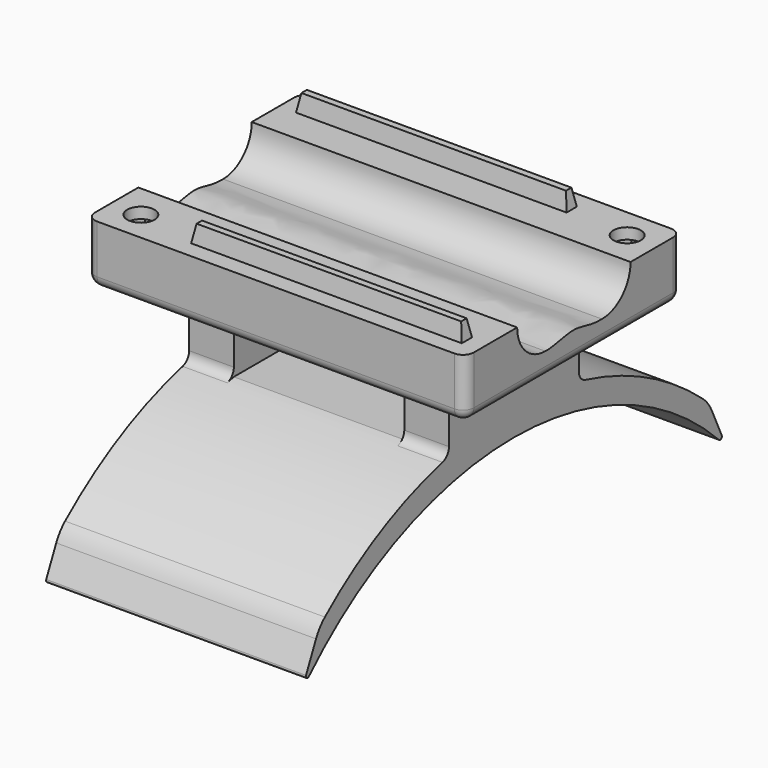
from build123d import *

# Parameters (mm, degrees)
F1_W          = 44.45
F1_H          = 31.75
F2_DEPTH      = 6.985
F4_DEPTH      = 44.45
F6_DEPTH      = 15.24
F6_DEPTH_BACK = 15.24
F7_W          = 20
F7_H          = 8.0811108913
F8_DEPTH      = 25.4
F9_R          = 1.6
F10_DEPTH     = 25.4
F11_R         = 1.6
F12_DEPTH     = 5.7
F13_W         = 31.75
F13_H         = 1.5
F14_DEPTH     = 2
F14_TAPER     = 10
F15_F1_R      = 0.254
F15_F2_R      = 0.254
F16_R         = 5.08
F18_R         = 1.27
F19_T1_DEPTH  = 5.24
F19_T3_DEPTH  = 5.24
F19_T5_DEPTH  = 8.89
F19_T7_DEPTH  = 29.21
F19_T9_DEPTH  = 41.91
F19_S13_W     = 1.2954
F19_S13_H     = 1.2954
F19_T14_DEPTH = 1.2954
F19_S19_W     = 1.2954
F19_S19_H     = 1.2954
F19_T20_DEPTH = 1.2954
F19_S25_W     = 1.2954
F19_S25_H     = 1.2954
F19_T26_DEPTH = 1.2954
F19_S31_W     = 1.2954
F19_S31_H     = 1.2954
F19_T32_DEPTH = 1.2954


# Not quite as in the source:
# - a fillet or chamfer that OpenCascade refuses, or shapes differently, is made with other operations: its cross-section is extruded or revolved along the edge and cut away or added
# - a feature of the source that left no trace in its solid (it failed there, or was rolled back) is left out


with BuildPart() as f2:
    # F1 (on Top) → F2 (new body)
    with BuildSketch(Plane.XY):
        Rectangle(F1_W, F1_H)
    extrude(amount=-F2_DEPTH)

    # F3 (on face) → F4 (cut, through all)
    with BuildSketch(Plane.YZ.offset(22.225)):
        with BuildLine():
            add(Edge.make_bspline(
                [(-4.125, 4.125), (-2.4255892558, 4.1137489608), (-0.0276085061, 2.971292738), (2.5249406681, 4.1137612248), (4.191, 4.191)],
                knots=[0, 0, 0, 0, 0.4977710734, 1, 1, 1, 1], degree=3))
            ThreePointArc((-4.125, 4.125), (-7.0418154724, 2.9168154724), (-8.25, 0))
            ThreePointArc((-8.25, 0), (-7.0418154724, -2.9168154724), (-4.125, -4.125))
            add(Edge.make_bspline(
                [(-4.125, -4.125), (-2.9335741419, -4.2006121948), (0.4172014685, -3.0581585459), (2.1438994445, -4.2006121948), (4.191, -4.191)],
                knots=[0, 0, 0, 0, 0.497799261, 1, 1, 1, 1], degree=3))
            ThreePointArc((4.191, -4.191), (7.15448452, -2.96348452), (8.382, 0))
            ThreePointArc((8.382, 0), (7.15448452, 2.96348452), (4.191, 4.191))
        make_face()
    extrude(amount=-F4_DEPTH, mode=Mode.SUBTRACT)

    # F5 (on Right) → F6 (join, two sides)
    with BuildSketch(Plane.YZ) as f6_sk:
        with BuildLine():
            ThreePointArc((-31.115, -30.5349261659), (0, -16.985), (31.115, -30.5349261659))
            Line((31.115, -30.5349261659), (28.575, -25.0251942949))
            ThreePointArc((28.575, -25.0251942949), (19.6900567688, -18.8213349574), (9.525, -15.0661108913))
            ThreePointArc((9.525, -15.0661108913), (0, -13.985), (-9.525, -15.0661108913))
            ThreePointArc((-9.525, -15.0661108913), (-19.6900567688, -18.8213349574), (-28.575, -25.0251942949))
            Line((-28.575, -25.0251942949), (-31.115, -30.5349261659))
        make_face()
        with BuildLine():
            ThreePointArc((-9.525, -15.0661108913), (0, -13.985), (9.525, -15.0661108913))
            Line((9.525, -15.0661108913), (9.525, -6.985))
            Line((9.525, -6.985), (-9.525, -6.985))
            Line((-9.525, -6.985), (-9.525, -15.0661108913))
        make_face()
    extrude(amount=F6_DEPTH)
    extrude(f6_sk.sketch, amount=-F6_DEPTH_BACK)

    # F7 (on face) → F8 (cut)
    with BuildSketch(Plane.XZ.offset(9.525)):
        with Locations((0, -11.0255554456)):
            Rectangle(F7_W, F7_H)
    extrude(amount=-F8_DEPTH, mode=Mode.SUBTRACT)

    # F9 (on face) → F10 (cut)
    with BuildSketch(Plane(origin=(0, 0, -6.985), x_dir=(1, 0, 0), z_dir=(0, 0, -1))):
        with Locations((-18.669, 12.319)):
            Circle(F9_R)
        with Locations((18.669, -12.319)):
            Circle(F9_R)
    extrude(amount=-F10_DEPTH, mode=Mode.SUBTRACT)

    # F11 (on face) → F12 (cut)
    with BuildSketch(Plane(origin=(0, 0, -6.985), x_dir=(1, 0, 0), z_dir=(0, 0, -1))):
        Polygon((-17.344, 10.02403268), (-16.019, 12.319), (-17.344, 14.61396732), (-19.994, 14.61396732), (-21.319, 12.319), (-19.994, 10.02403268), align=None)
        with Locations((-18.669, 12.319)):
            Circle(F11_R, mode=Mode.SUBTRACT)
        Polygon((19.994, -14.61396732), (21.319, -12.319), (19.994, -10.02403268), (17.344, -10.02403268), (16.019, -12.319), (17.344, -14.61396732), align=None)
        with Locations((18.669, -12.319)):
            Circle(F11_R, mode=Mode.SUBTRACT)
    extrude(amount=-F12_DEPTH, mode=Mode.SUBTRACT)

    # F13 (on face) → F14 (join)
    with BuildSketch(Plane.XY):
        with Locations((-4.35, 13.125)):
            Rectangle(F13_W, F13_H)
        with Locations((4.35, -13.125)):
            Rectangle(F13_W, F13_H)
    extrude(amount=F14_DEPTH, taper=F14_TAPER)

    # F15: fillet of radius 0.254 on 2 edges, made by hand

    # F15_f1
    f15_f1_edges = [f2.edges().sort_by_distance(p)[0] for p in [
        (0, -31.115, -30.5349261659),
    ]]
    fillet(f15_f1_edges, radius=F15_F1_R)

    # F15_f2
    f15_f2_edges = [f2.edges().sort_by_distance(p)[0] for p in [
        (0, 31.115, -30.5349261659),
    ]]
    fillet(f15_f2_edges, radius=F15_F2_R)

    # F16
    f16_edges = [f2.edges().sort_by_distance(p)[0] for p in [
        (0, 28.575, -25.025194),
        (0, -28.575, -25.025194),
    ]]
    fillet(f16_edges, radius=F16_R)

    # F18
    f18_edges = [f2.edges().sort_by_distance(p)[0] for p in [
        (12.62, 9.525, -6.985),
        (15.24, 0, -6.985),
        (12.62, -9.525, -6.985),
        (10, 0, -6.985),
        (-12.62, -9.525, -6.985),
        (-15.24, 0, -6.985),
        (-10, 0, -6.985),
        (-12.62, 9.525, -6.985),
    ]]
    fillet(f18_edges, radius=F18_R)

    # F19: fillet of radius 1.27 on 12 edges, made by hand

    # F19_s2 → F19_t1 (join)
    with BuildSketch(Plane.YZ.offset(-15.24)):
        with BuildLine():
            ThreePointArc((9.525, -14.0670689448), (9.7923311345, -14.8465271838), (10.4817797578, -15.2978382489))
            ThreePointArc((10.4817797578, -15.2978382489), (10.0040608486, -15.1792042016), (9.525, -15.0661108913))
            Line((9.525, -15.0661108913), (9.525, -14.0670689448))
        make_face()
        with BuildLine():
            ThreePointArc((-9.525, -14.0670689448), (-9.7923311345, -14.8465271838), (-10.4817797578, -15.2978382489))
            ThreePointArc((-10.4817797578, -15.2978382489), (-10.0040608486, -15.1792042016), (-9.525, -15.0661108913))
            Line((-9.525, -15.0661108913), (-9.525, -14.0670689448))
        make_face()
    extrude(amount=F19_T1_DEPTH)

    # F19_s4 → F19_t3 (join)
    with BuildSketch(Plane.YZ.offset(10)):
        with BuildLine():
            ThreePointArc((10.4817797578, -15.2978382489), (9.7923311345, -14.8465271838), (9.525, -14.0670689448))
            Line((9.525, -14.0670689448), (9.525, -15.0661108913))
            ThreePointArc((9.525, -15.0661108913), (10.0040608486, -15.1792042016), (10.4817797578, -15.2978382489))
        make_face()
        with BuildLine():
            ThreePointArc((-10.4817797578, -15.2978382489), (-9.7923311345, -14.8465271838), (-9.525, -14.0670689448))
            Line((-9.525, -14.0670689448), (-9.525, -15.0661108913))
            ThreePointArc((-9.525, -15.0661108913), (-10.0040608486, -15.1792042016), (-10.4817797578, -15.2978382489))
        make_face()
    extrude(amount=F19_T3_DEPTH)

    # F19_s6 → F19_t5 (cut)
    with BuildSketch(Plane.XY.offset(-5.715)):
        with BuildLine():
            ThreePointArc((-20.955, -15.875), (-21.8530256121, -15.5030256121), (-22.225, -14.605))
            Line((-22.225, -14.605), (-22.225, -15.875))
            Line((-22.225, -15.875), (-20.955, -15.875))
        make_face()
        with BuildLine():
            ThreePointArc((22.225, -14.605), (21.8530256121, -15.5030256121), (20.955, -15.875))
            Line((20.955, -15.875), (22.225, -15.875))
            Line((22.225, -15.875), (22.225, -14.605))
        make_face()
        with BuildLine():
            ThreePointArc((22.225, 14.605), (21.8530256121, 15.5030256121), (20.955, 15.875))
            Line((20.955, 15.875), (22.225, 15.875))
            Line((22.225, 15.875), (22.225, 14.605))
        make_face()
        with BuildLine():
            ThreePointArc((-20.955, 15.875), (-21.8530256121, 15.5030256121), (-22.225, 14.605))
            Line((-22.225, 14.605), (-22.225, 15.875))
            Line((-22.225, 15.875), (-20.955, 15.875))
        make_face()
    extrude(amount=F19_T5_DEPTH, mode=Mode.SUBTRACT)

    # F19_s8 → F19_t7 (cut)
    with BuildSketch(Plane.XZ.offset(-14.605)):
        with BuildLine():
            ThreePointArc((-20.955, -6.985), (-21.8530256121, -6.6130256121), (-22.225, -5.715))
            Line((-22.225, -5.715), (-22.225, -6.985))
            Line((-22.225, -6.985), (-20.955, -6.985))
        make_face()
        with BuildLine():
            ThreePointArc((20.955, -6.985), (21.8530256121, -6.6130256121), (22.225, -5.715))
            Line((22.225, -5.715), (22.225, -6.985))
            Line((22.225, -6.985), (20.955, -6.985))
        make_face()
    extrude(amount=F19_T7_DEPTH, mode=Mode.SUBTRACT)

    # F19_s10 → F19_t9 (cut)
    with BuildSketch(Plane.YZ.offset(-20.955)):
        with BuildLine():
            ThreePointArc((-14.605, -6.985), (-15.5030256121, -6.6130256121), (-15.875, -5.715))
            Line((-15.875, -5.715), (-15.875, -6.985))
            Line((-15.875, -6.985), (-14.605, -6.985))
        make_face()
        with BuildLine():
            ThreePointArc((14.605, -6.985), (15.5030256121, -6.6130256121), (15.875, -5.715))
            Line((15.875, -5.715), (15.875, -6.985))
            Line((15.875, -6.985), (14.605, -6.985))
        make_face()
    extrude(amount=F19_T9_DEPTH, mode=Mode.SUBTRACT)


with BuildPart() as f19_tool12:
    # F19_s13 → F19_t14 (new body)
    with BuildSketch(Plane.YZ.offset(-20.955)):
        with Locations((-15.2527, -6.3627)):
            Rectangle(F19_S13_W, F19_S13_H)
    extrude(amount=-F19_T14_DEPTH)

    # F19_s15 → F19_t16 (revolve, cut)
    with BuildSketch(Plane(origin=(-20.955, -14.605, -5.715), x_dir=(0, 0.7071067812, 0.7071067812), z_dir=(0, -0.7071067812, 0.7071067812))):
        with BuildLine():
            ThreePointArc((0, -1.27), (1.27, 0), (0, 1.27))
            Line((0, 1.27), (0, -1.27))
        make_face()
    revolve(axis=Axis((-20.955, -14.605, -5.715), (-1, 0, 0)), mode=Mode.SUBTRACT)


with BuildPart() as f2_1:
    add(f2.part)

    # F19_t11: cut F19_tool12
    add(f19_tool12.part, mode=Mode.SUBTRACT)


with BuildPart() as f19_tool18:
    # F19_s19 → F19_t20 (new body)
    with BuildSketch(Plane.XY.offset(-5.715)):
        with Locations((-21.6027, 15.2527)):
            Rectangle(F19_S19_W, F19_S19_H)
    extrude(amount=-F19_T20_DEPTH)

    # F19_s21 → F19_t22 (revolve, cut)
    with BuildSketch(Plane(origin=(-20.955, 14.605, -5.715), x_dir=(0.7071067812, -0.7071067812, 0), z_dir=(0.7071067812, 0.7071067812, 0))):
        with BuildLine():
            ThreePointArc((0, -1.27), (1.27, 0), (0, 1.27))
            Line((0, 1.27), (0, -1.27))
        make_face()
    revolve(axis=Axis((-20.955, 14.605, -5.715), (0, 0, -1)), mode=Mode.SUBTRACT)


with BuildPart() as f2_2:
    add(f2_1.part)

    # F19_t17: cut F19_tool18
    add(f19_tool18.part, mode=Mode.SUBTRACT)


with BuildPart() as f19_tool24:
    # F19_s25 → F19_t26 (new body)
    with BuildSketch(Plane.XY.offset(-5.715)):
        with Locations((21.6027, -15.2527)):
            Rectangle(F19_S25_W, F19_S25_H)
    extrude(amount=-F19_T26_DEPTH)

    # F19_s27 → F19_t28 (revolve, cut)
    with BuildSketch(Plane(origin=(20.955, -14.605, -5.715), x_dir=(-0.7071067812, 0.7071067812, 0), z_dir=(-0.7071067812, -0.7071067812, 0))):
        with BuildLine():
            ThreePointArc((0, -1.27), (1.27, 0), (0, 1.27))
            Line((0, 1.27), (0, -1.27))
        make_face()
    revolve(axis=Axis((20.955, -14.605, -5.715), (0, 0, -1)), mode=Mode.SUBTRACT)


with BuildPart() as f2_3:
    add(f2_2.part)

    # F19_t23: cut F19_tool24
    add(f19_tool24.part, mode=Mode.SUBTRACT)


with BuildPart() as f19_tool30:
    # F19_s31 → F19_t32 (new body)
    with BuildSketch(Plane.XY.offset(-5.715)):
        with Locations((21.6027, 15.2527)):
            Rectangle(F19_S31_W, F19_S31_H)
    extrude(amount=-F19_T32_DEPTH)

    # F19_s33 → F19_t34 (revolve, cut)
    with BuildSketch(Plane(origin=(20.955, 14.605, -5.715), x_dir=(-0.7071067812, -0.7071067812, 0), z_dir=(0.7071067812, -0.7071067812, 0))):
        with BuildLine():
            ThreePointArc((0, -1.27), (1.27, 0), (0, 1.27))
            Line((0, 1.27), (0, -1.27))
        make_face()
    revolve(axis=Axis((20.955, 14.605, -5.715), (0, 0, -1)), mode=Mode.SUBTRACT)


with BuildPart() as f2_4:
    add(f2_3.part)

    # F19_t29: cut F19_tool30
    add(f19_tool30.part, mode=Mode.SUBTRACT)


solid = f2_4.part
